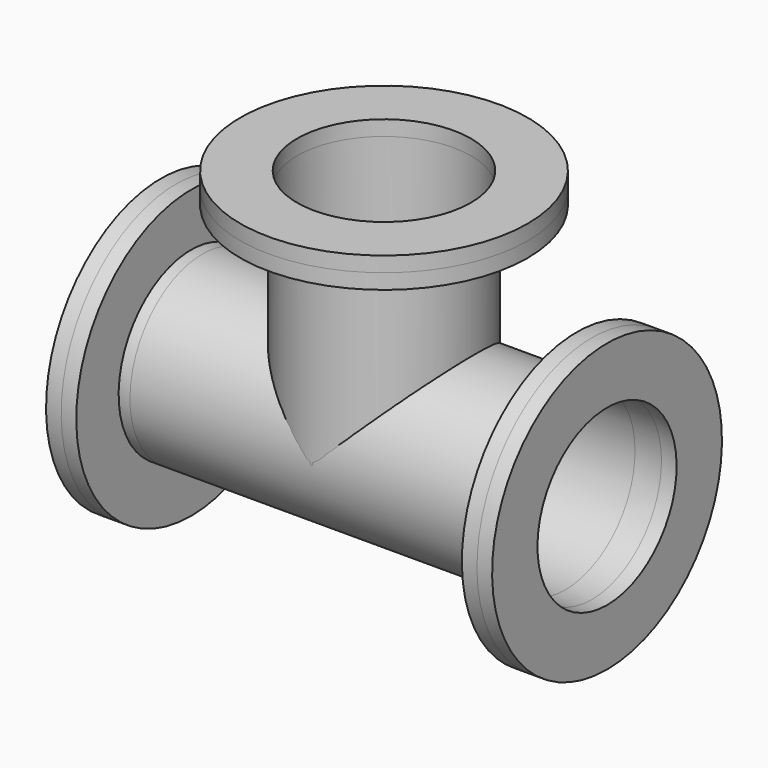
from build123d import *

# Parameters (mm, degrees)
F0_R      = 152.4
F0_R_2    = 146.05
F1_DEPTH  = 19.05
F2_R      = 241.3
F2_R_2    = 152.4
F2_R_3    = 146.05
F3_DEPTH  = 25.4
F9_ANGLE  = 90
F11_DEPTH = 609.6
F12_REACH = 977.1532938113
F13_DEPTH = 25.4
F14_DEPTH = 25.4
F15_DEPTH = 25.4


with BuildPart() as f1:
    # F0 (on Top) → F1 (new body)
    with BuildSketch(Plane.XY):
        Circle(F0_R)
        Circle(F0_R_2, mode=Mode.SUBTRACT)
    extrude(amount=F1_DEPTH)

    # F2 (on face) → F3 (join)
    with BuildSketch(Plane.XY.offset(19.05)):
        Circle(F2_R)
        Circle(F2_R_2, mode=Mode.SUBTRACT)
        Circle(F2_R_2)
        Circle(F2_R_3, mode=Mode.SUBTRACT)
    extrude(amount=F3_DEPTH)


with BuildPart() as f7_1:
    # F7: copy of F1
    add(f1.part.moved(Location((304.8, 0, -304.8))))


with BuildPart() as f7_1_1:
    # F9: moved
    add(f7_1.part.rotate(Axis((304.8, 122.1911609173, -304.8), (0, 1, 0)), F9_ANGLE))


with BuildPart() as f10_1:
    # F10: instance of F7_1
    add(f7_1_1.part.mirror(Plane.YZ))


with BuildPart() as f7_1_2:
    add(f7_1_1.part)

    # F11 (add, through all): a face of the model
    f11_faces = [f7_1_2.faces().sort_by_distance(p)[0] for p in [
        (304.8, 0, -156.7105229381),
    ]]

    add(f10_1.part)  # F11 merges F10_1
    extrude(f11_faces, amount=F11_DEPTH)


with BuildPart() as f1_1:
    add(f1.part)

    f12_end = f7_1_2.part.faces().sort_by_distance((0, 0, -152.4))[0]
    # F0 (on Top) → F12 (join, up to a face of F7_1 that its end follows)
    with BuildSketch(Plane.XY):
        Circle(F0_R)
        Circle(F0_R_2, mode=Mode.SUBTRACT)
    f12_long = extrude(amount=-F12_REACH, mode=Mode.PRIVATE)
    add(split(f12_long, bisect_by=f12_end, keep=Keep.ALL, mode=Mode.PRIVATE).solids().sort_by_distance((-148.0894770619, 0, 0))[0])


with BuildPart() as f13:
    # F13 (new): a face of the model
    f13_faces = [f7_1_2.part.faces().sort_by_distance(p)[0] for p in [
        (349.25, 0, -70.324994652),
    ]]
    extrude(f13_faces, amount=F13_DEPTH)


with BuildPart() as f14:
    # F14 (new): a face of the model
    f14_faces = [f7_1_2.part.faces().sort_by_distance(p)[0] for p in [
        (-349.25, 0, -70.324994652),
    ]]
    extrude(f14_faces, amount=F14_DEPTH)


with BuildPart() as f15:
    # F15 (new): a face of the model
    f15_faces = [f1_1.part.faces().sort_by_distance(p)[0] for p in [
        (-234.475005348, 0, 44.45),
    ]]
    extrude(f15_faces, amount=F15_DEPTH)


solid = Compound([f7_1_2.part, f1_1.part, f13.part, f14.part, f15.part])
